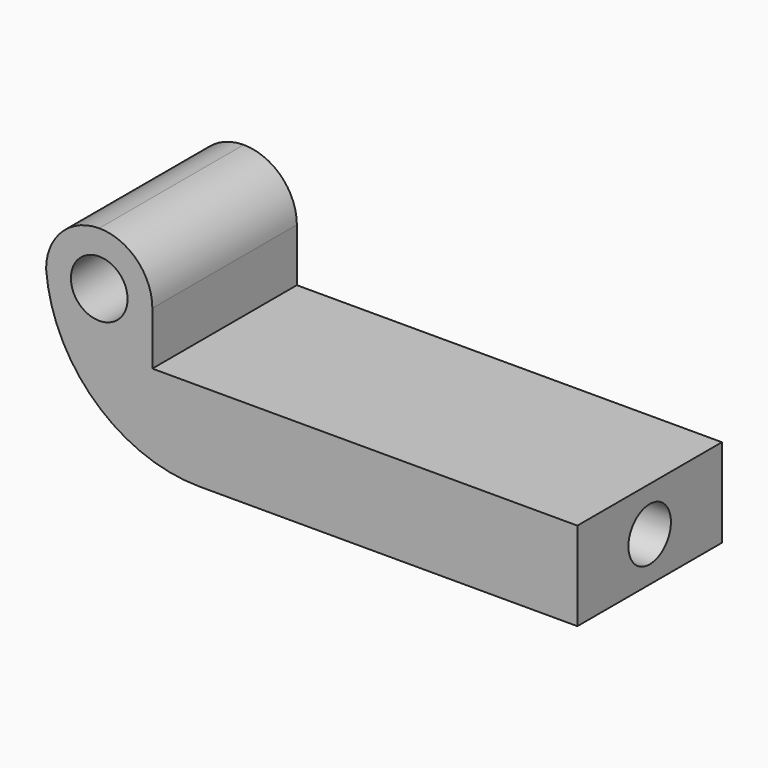
from build123d import *

# Parameters (mm, degrees)
F0_W        = 30
F0_H        = 10.2
F0_W_2      = 7.5
F0_H_2      = 9.8
F1_DEPTH    = 5
F2_W        = 6
F2_H        = 10.2
F3_DEPTH    = 6
F4_R        = 1.6
F5_DEPTH    = 25
F6_R        = 2.99999
F7_T1_DEPTH = 53.5182164383
F8_R        = 1.5
F9_DEPTH    = 7


# Not quite as in the source:
# - a fillet or chamfer that OpenCascade refuses, or shapes differently, is made with other operations: its cross-section is extruded or revolved along the edge and cut away or added
# - a fillet or chamfer is up to 0.001 mm smaller than in the source, because OpenCascade refuses the exact size


with BuildPart() as f1:
    # F0 (on Top) → F1 (new body)
    with BuildSketch(Plane.XY):
        Rectangle(F0_W, F0_H)
        with Locations((7.25, 0)):
            Rectangle(F0_W_2, F0_H_2, mode=Mode.SUBTRACT)
        with Locations((7.25, 0)):
            Rectangle(F0_W_2, F0_H_2)
    extrude(amount=F1_DEPTH)

    # F2 (on face) → F3 (join)
    with BuildSketch(Plane.XY.offset(5)):
        with Locations((-12, 0)):
            Rectangle(F2_W, F2_H)
    extrude(amount=F3_DEPTH)

    # F4 (on face) → F5 (cut)
    with BuildSketch(Plane.XZ.offset(5.1)):
        with Locations((-12, 8)):
            Circle(F4_R)
    extrude(amount=-F5_DEPTH, mode=Mode.SUBTRACT)

    # F6 (radius 3 in the source; OpenCascade refuses exactly that, so slightly less here)
    f6_edges = [f1.edges().sort_by_distance(p)[0] for p in [
        (-9, 0, 11),
        (-15, 0, 11),
    ]]
    fillet(f6_edges, radius=F6_R)

    # F7: fillet of radius 8.6911688245 on 1 edges, made by hand

    # F7_s2 → F7_t1 (cut)
    with BuildSketch(Plane.XZ.offset(-26.7591082192)):
        with BuildLine():
            ThreePointArc((-15, 8.00001), (-12.2325180699, 2.3058969601), (-6.3363567123, 0))
            Line((-6.3363567123, 0), (-6.3363567123, -0.1738233765))
            Line((-6.3363567123, -0.1738233765), (-15, -0.1738233765))
            Line((-15, -0.1738233765), (-15.1738233765, 0))
            ThreePointArc((-15.1738233765, 0), (-15.1738233765, 4.000005), (-15.1732728658, 7.9861868235))
            Line((-15.1732728658, 7.9861868235), (-15, 8.00001))
        make_face()
    extrude(amount=F7_T1_DEPTH, mode=Mode.SUBTRACT)

    # F8 (on face) → F9 (cut)
    with BuildSketch(Plane.YZ.offset(15)):
        with Locations((0, 2.5)):
            Circle(F8_R)
    extrude(amount=-F9_DEPTH, mode=Mode.SUBTRACT)


solid = f1.part
